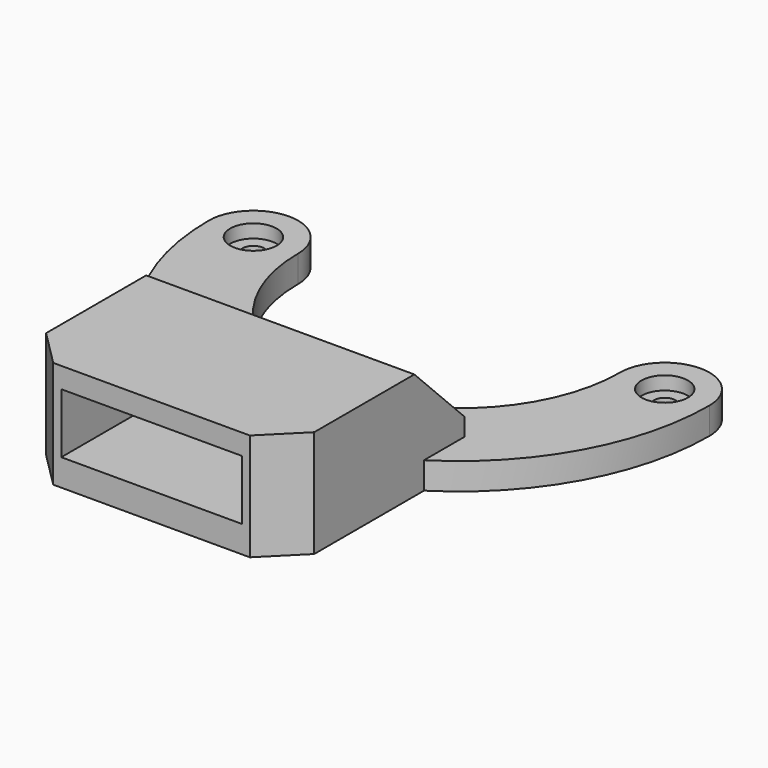
from build123d import *

# Parameters (mm, degrees)
F1_DEPTH       = 3
F2_R           = 4.99999
F4_D           = 2.4384
F4_CBORE_D     = 5.2
F4_CBORE_DEPTH = 1.5
F5_W           = 30
F5_H           = 25
F6_DEPTH       = 12
F8_DEPTH       = 25.001
F9_T1_DEPTH    = 66.0035618315
F10_SIZE       = 4


# Not quite as in the source:
# - a fillet or chamfer that OpenCascade refuses, or shapes differently, is made with other operations: its cross-section is extruded or revolved along the edge and cut away or added
# - a fillet or chamfer is up to 0.001 mm smaller than in the source, because OpenCascade refuses the exact size


with BuildPart() as f1:
    # F0 (on Top) → F1 (new body)
    with BuildSketch(Plane.XY):
        with BuildLine():
            ThreePointArc((18.0125, 0), (0, -18.0125), (-18.0125, 0))
            Line((-18.0125, 0), (-18.0125, 5))
            Line((-18.0125, 5), (-28.0125, 5))
            Line((-28.0125, 5), (-28.0125, 0))
            ThreePointArc((-28.0125, 0), (0, -28.0125), (28.0125, 0))
            Line((28.0125, 0), (28.0125, 5))
            Line((28.0125, 5), (18.0125, 5))
            Line((18.0125, 5), (18.0125, 0))
        make_face()
    extrude(amount=F1_DEPTH)

    # F2 (radius 5 in the source; OpenCascade refuses exactly that, so slightly less here)
    f2_edges = [f1.edges().sort_by_distance(p)[0] for p in [
        (-28.0125, 5, 1.5),
        (-18.0125, 5, 1.5),
        (18.0125, 5, 1.5),
        (28.0125, 5, 1.5),
    ]]
    fillet(f2_edges, radius=F2_R)

    # F4 (through all)
    with Locations(Plane.XY.offset(3)):
        with Locations((-23.0125, 0), (23.0125, 0)):
            CounterBoreHole(F4_D / 2, F4_CBORE_D / 2, F4_CBORE_DEPTH)

    # F5 (on Top) → F6 (join)
    with BuildSketch(Plane.XY):
        with Locations((0, -30.5125)):
            Rectangle(F5_W, F5_H)
    extrude(amount=F6_DEPTH)

    # F7 (on face) → F8 (cut, through all)
    with BuildSketch(Plane(origin=(0, -18.0125, 0), x_dir=(-1, 0, 0), z_dir=(0, 1, 0))):
        Polygon((0, 3), (10.1, 3), (10.1, 9.7), (-10.1, 9.7), (-10.1, 3), align=None)
    extrude(amount=-F8_DEPTH, mode=Mode.SUBTRACT)

    # F9: chamfer of 7 on 1 edges, made by hand

    # F9_s2 → F9_t1 (cut)
    with BuildSketch(Plane.YZ.offset(-33.0017809158)):
        Polygon((-25.0125, 12), (-18.0125, 5), (-18.0125, 12), align=None)
    extrude(amount=F9_T1_DEPTH, mode=Mode.SUBTRACT)

    # F10
    f10_edges = [f1.edges().sort_by_distance(p)[0] for p in [
        (-15, -43.0125, 6),
        (15, -43.0125, 6),
    ]]
    chamfer(f10_edges, length=F10_SIZE)


solid = f1.part
